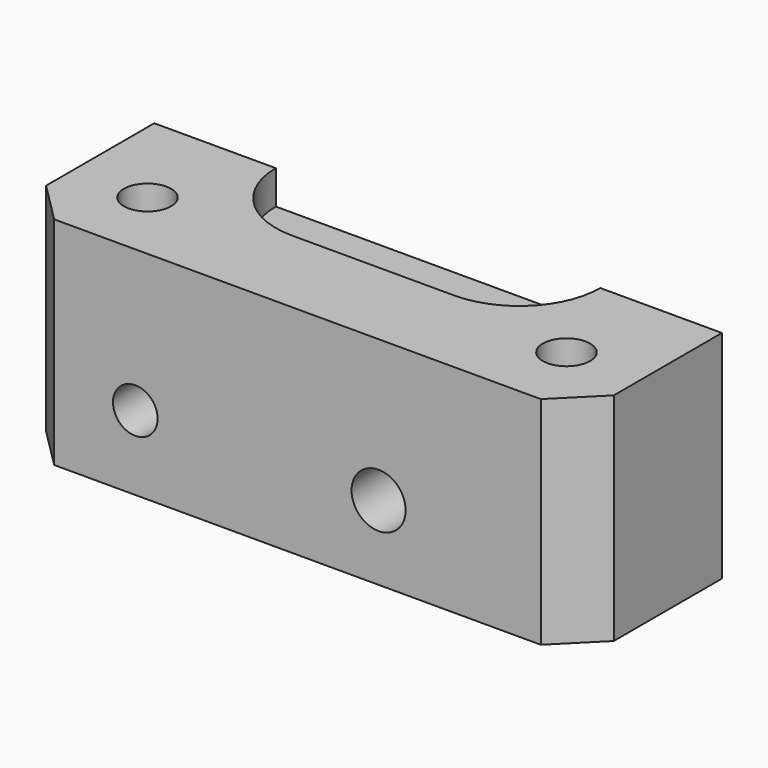
from build123d import *

# Parameters (mm, degrees)
F0_W     = 42
F0_H     = 13
F0_R     = 1.75
F1_DEPTH = 8
F2_W     = 24
F2_H     = 6
F3_DEPTH = 2.5
F4_R     = 5.99999
F5_SIZE  = 3
F6_R     = 1.65
F6_R_2   = 2
F7_DEPTH = 13.001


# Not quite as in the source:
# - a fillet or chamfer is up to 0.001 mm smaller than in the source, because OpenCascade refuses the exact size


with BuildPart() as f1:
    # F0 (on Top) → F1 (new body, symmetric)
    with BuildSketch(Plane.XY):
        Rectangle(F0_W, F0_H)
        with Locations((-15.5, -1)):
            Circle(F0_R, mode=Mode.SUBTRACT)
        with Locations((15.5, -1)):
            Circle(F0_R, mode=Mode.SUBTRACT)
    extrude(amount=F1_DEPTH, both=True)

    # F2 (on face) → F3 (cut)
    with BuildSketch(Plane.XY.offset(8)):
        with Locations((0, 3.5)):
            Rectangle(F2_W, F2_H)
    extrude(amount=-F3_DEPTH, mode=Mode.SUBTRACT)

    # F4 (radius 6 in the source; OpenCascade refuses exactly that, so slightly less here)
    f4_edges = [f1.edges().sort_by_distance(p)[0] for p in [
        (-12, 0.5, 6.75),
        (12, 0.5, 6.75),
    ]]
    fillet(f4_edges, radius=F4_R)

    # F5
    f5_edges = [f1.edges().sort_by_distance(p)[0] for p in [
        (-21, -6.5, 0),
        (21, -6.5, 0),
    ]]
    chamfer(f5_edges, length=F5_SIZE)

    # F6 (on face) → F7 (cut, through all)
    with BuildSketch(Plane(origin=(0, 6.5, 0), x_dir=(-1, 0, 0), z_dir=(0, 1, 0))):
        with Locations((12, -2.5)):
            Circle(F6_R)
        with Locations((-6, -2.5)):
            Circle(F6_R_2)
    extrude(amount=-F7_DEPTH, mode=Mode.SUBTRACT)


solid = f1.part
